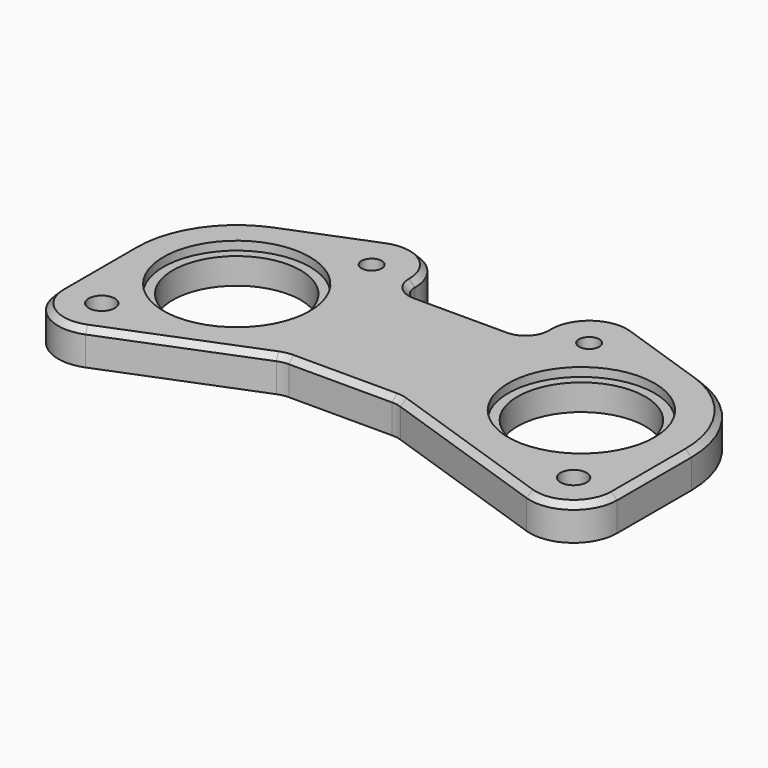
from build123d import *

# Parameters (mm, degrees)
F0_R     = 4.5
F0_R_2   = 22
F0_R_3   = 3.5
F1_DEPTH = 12
F2_R     = 25.2
F3_DEPTH = 3
F4_SIZE  = 2
F5_R     = 30.5
F5_R_2   = 27.5
F6_DEPTH = 2.5


# Not quite as in the source:
# - ends of sketch curves that miss each other by under 0.0002 mm in the source are joined


with BuildPart() as f1:
    # F0 (on Top) → F1 (new body)
    with BuildSketch(Plane.XY):
        with BuildLine():
            Line((-96.25, -7.835472), (-96.25, -39.300472))
            ThreePointArc((-96.25, -39.300472), (-89.6603385796, -51.720866719), (-75.6811726698, -53.2284353172))
            Line((-75.6811726698, -53.2284353172), (-25.901923657, -33.3251628629))
            ThreePointArc((-25.901923657, -33.3251628629), (-24.0797305928, -32.7907701516), (-22.189372, -32.610472))
            Line((-22.189372, -32.610472), (13.41096, -32.610472))
            ThreePointArc((13.41096, -32.610472), (15.0445629213, -32.7448072228), (16.6342757601, -33.1442037009))
            Line((16.6342757601, -33.1442037009), (76.4150264593, -53.4998741564))
            ThreePointArc((76.4150264593, -53.4998741564), (89.9814201421, -51.4972872524), (96.25, -39.300472))
            Line((96.25, -39.300472), (96.25, -7.385472))
            ThreePointArc((96.25, -7.385472), (89.1771507076, 14.6451910108), (70.602136617, 28.4417181588))
            Line((70.602136617, 28.4417181588), (40.3905414757, 38.7289301785))
            ThreePointArc((40.3905414757, 38.7289301785), (26.82414783, 36.7263432324), (20.555568, 24.529528))
            Line((20.555568, 24.529528), (20.555568, 23.389528))
            ThreePointArc((20.555568, 23.389528), (18.7982086871, 19.1468873129), (14.555568, 17.389528))
            Line((14.555568, 17.389528), (-17.637618, 17.389528))
            ThreePointArc((-17.637618, 17.389528), (-21.8802586871, 19.1468873129), (-23.637618, 23.389528))
            Line((-23.637618, 23.389528), (-23.637618, 23.629528))
            ThreePointArc((-23.637618, 23.629528), (-30.2272793638, 36.0499226807), (-44.2064452032, 37.557491368))
            Line((-44.2064452032, 37.557491368), (-73.4226694122, 25.875948235))
            ThreePointArc((-73.4226694122, 25.875948235), (-90.0062904382, 12.5210187268), (-96.25, -7.835472))
        make_face()
        with Locations((-81.25, -39.300472)):
            Circle(F0_R, mode=Mode.SUBTRACT)
        with Locations((-59.943809, -7.835472)):
            Circle(F0_R_2, mode=Mode.SUBTRACT)
        with Locations((81.25, -39.300472)):
            Circle(F0_R, mode=Mode.SUBTRACT)
        with Locations((-38.637618, 23.629528)):
            Circle(F0_R_3, mode=Mode.SUBTRACT)
        with Locations((58.402784, -7.385472)):
            Circle(F0_R_2, mode=Mode.SUBTRACT)
        with Locations((35.555568, 24.529528)):
            Circle(F0_R_3, mode=Mode.SUBTRACT)
    extrude(amount=F1_DEPTH)

    # F2 (on face) → F3 (cut)
    with BuildSketch(Plane.XY.offset(12)):
        with Locations((-59.943809, -7.835472)):
            Circle(F2_R)
        with Locations((58.402784, -7.385472)):
            Circle(F2_R)
    extrude(amount=-F3_DEPTH, mode=Mode.SUBTRACT)

    # F4
    f4_edges = [f1.edges().sort_by_distance(p)[0] for p in [
        (-58.814557, 31.71672, 12),
    ]]
    chamfer(f4_edges, length=F4_SIZE)

    # F5 (on face) → F6 (cut)
    with BuildSketch(Plane(origin=(0, 0, 0), x_dir=(1, 0, 0), z_dir=(0, 0, -1))):
        with Locations((-59.943809, 7.835472)):
            Circle(F5_R)
        with Locations((-59.943809, 7.835472)):
            Circle(F5_R_2, mode=Mode.SUBTRACT)
        with Locations((58.402784, 7.385472)):
            Circle(F5_R)
        with Locations((58.402784, 7.385472)):
            Circle(F5_R_2, mode=Mode.SUBTRACT)
    extrude(amount=-F6_DEPTH, mode=Mode.SUBTRACT)


solid = f1.part
